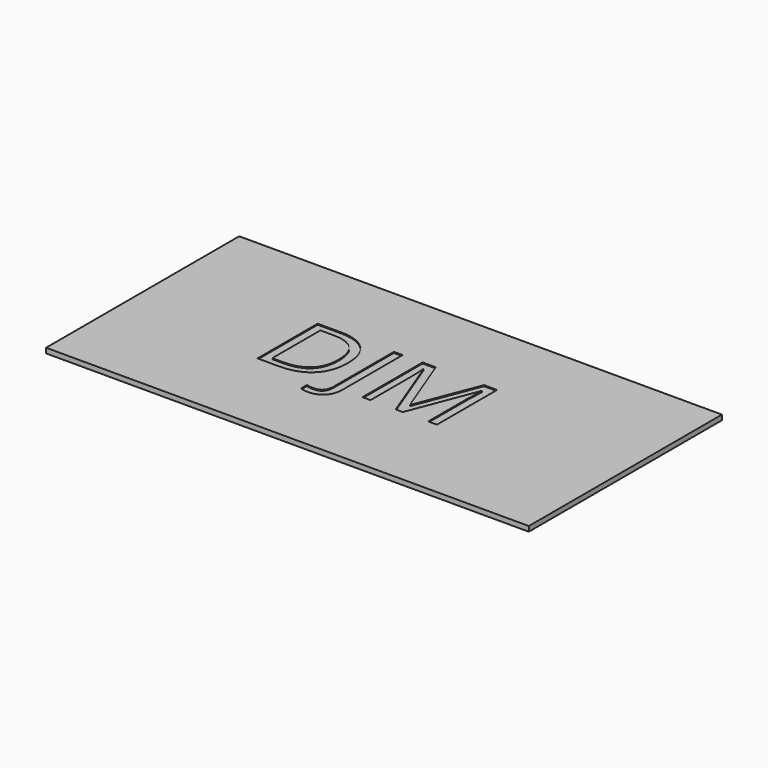
from build123d import *

# Parameters (mm, degrees)
F0_W         = 304.8
F0_H         = 152.4
F1_DEPTH     = 3.175
F2_TEXT_SIZE = 66.5156895088
F3_DEPTH     = 0.635


# Not quite as in the source:
# - Text() gives the source's letters only with a copy of the font that has no kerning and outlines rounded to 1/6400 em; it was checked with that copy


with BuildPart() as f1:
    # F0 (on Top) → F1 (new body)
    with BuildSketch(Plane.XY):
        with Locations((86.8385266513, -65.443836686)):
            Rectangle(F0_W, F0_H)
    extrude(amount=F1_DEPTH)

    # F2 (on face) → F3 (cut)
    with BuildSketch(Plane.XY.offset(3.175)):
        with Locations((16.4282415062, -85.4297056794)):
            Text('DJM', F2_TEXT_SIZE, font='Open Sans', text_align=(TextAlign.LEFT, TextAlign.BOTTOM))
    extrude(amount=-F3_DEPTH, mode=Mode.SUBTRACT)


solid = f1.part
